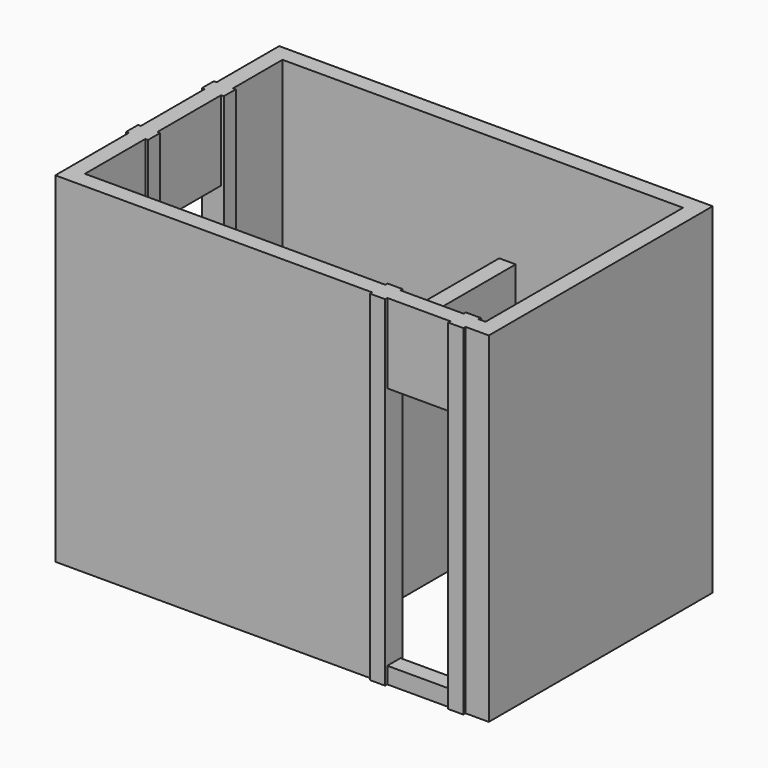
from build123d import *

# Parameters (mm, degrees)
F0_W     = 152.4
F0_H     = 139.7
F0_W_2   = 25.4
F0_W_3   = 139.7
F0_H_2   = 152.4
F0_H_3   = 25.4
F1_DEPTH = 2997.2
F2_START = 2260.6
F0_H_4   = 736.6
F0_W_4   = 584.2
F2_DEPTH = 736.6
F0_H_5   = 2286
F3_DEPTH = 152.4
F4_DEPTH = 2032


with BuildPart() as f1:
    # F0 (on Top) → F1 (new body)
    with BuildSketch(Plane.XY):
        Polygon((2006.6, 0), (0, 0), (0, 698.5), (-152.4, 698.5), (-152.4, -152.4), (2781.3, -152.4), (2781.3, 0), (2159, 0), align=None)
        with Locations((-76.2, 768.35)):
            Rectangle(F0_W, F0_H)
        with Locations((12.7, 768.35)):
            Rectangle(F0_W_2, F0_H)
        with Locations((-165.1, 768.35)):
            Rectangle(F0_W_2, F0_H)
        Polygon((2781.3, 25.4), (2781.3, 0), (2921, 0), (2921, 25.4), (2844.8, 25.4), align=None)
        with Locations((2851.15, -76.2)):
            Rectangle(F0_W_3, F0_H_2)
        with Locations((2851.15, -165.1)):
            Rectangle(F0_W_3, F0_H_3)
    extrude(amount=F1_DEPTH)



with BuildPart() as f1b:
    # F0 (on Top) → F1, piece 2 (new body)
    with BuildSketch(Plane.XY):
        Polygon((0, 2286), (2006.6, 2286), (2159, 2286), (3708.4, 2286), (3708.4, 0), (3644.9, 0), (3644.9, -152.4), (3860.8, -152.4), (3860.8, 2438.4), (-152.4, 2438.4), (-152.4, 1714.5), (0, 1714.5), align=None)
        with Locations((-76.2, 1644.65)):
            Rectangle(F0_W, F0_H)
        with Locations((12.7, 1644.65)):
            Rectangle(F0_W_2, F0_H)
        with Locations((-165.1, 1644.65)):
            Rectangle(F0_W_2, F0_H)
        with Locations((3575.05, 12.7)):
            Rectangle(F0_W_3, F0_H_3)
        with Locations((3575.05, -76.2)):
            Rectangle(F0_W_3, F0_H_2)
        with Locations((3575.05, -165.1)):
            Rectangle(F0_W_3, F0_H_3)
    extrude(amount=F1_DEPTH)


with BuildPart() as f1_1:
    add(f1.part)

    add(f1b.part)  # F2 merges F1b
    # F0 (on Top) → F2 (join)
    with BuildSketch(Plane.XY.offset(F2_START)):
        with Locations((-76.2, 1206.5)):
            Rectangle(F0_W, F0_H_4)
        with Locations((3213.1, -76.2)):
            Rectangle(F0_W_4, F0_H_2)
    extrude(amount=F2_DEPTH)

    # F0 (on Top) → F3 (join)
    with BuildSketch(Plane.XY):
        Polygon((2006.6, 0), (0, 0), (0, 698.5), (-152.4, 698.5), (-152.4, -152.4), (2781.3, -152.4), (2781.3, 0), (2159, 0), align=None)
        with Locations((2082.8, 1143)):
            Rectangle(F0_W, F0_H_5)
        with Locations((-76.2, 768.35)):
            Rectangle(F0_W, F0_H)
        with Locations((12.7, 768.35)):
            Rectangle(F0_W_2, F0_H)
        Polygon((0, 2286), (2006.6, 2286), (2159, 2286), (3708.4, 2286), (3708.4, 0), (3644.9, 0), (3644.9, -152.4), (3860.8, -152.4), (3860.8, 2438.4), (-152.4, 2438.4), (-152.4, 1714.5), (0, 1714.5), align=None)
        with Locations((-76.2, 1206.5)):
            Rectangle(F0_W, F0_H_4)
        with Locations((-165.1, 768.35)):
            Rectangle(F0_W_2, F0_H)
        Polygon((2781.3, 25.4), (2781.3, 0), (2921, 0), (2921, 25.4), (2844.8, 25.4), align=None)
        with Locations((2851.15, -76.2)):
            Rectangle(F0_W_3, F0_H_2)
        with Locations((-76.2, 1644.65)):
            Rectangle(F0_W, F0_H)
        with Locations((12.7, 1644.65)):
            Rectangle(F0_W_2, F0_H)
        with Locations((3213.1, -76.2)):
            Rectangle(F0_W_4, F0_H_2)
        with Locations((2851.15, -165.1)):
            Rectangle(F0_W_3, F0_H_3)
        with Locations((-165.1, 1644.65)):
            Rectangle(F0_W_2, F0_H)
        with Locations((3575.05, 12.7)):
            Rectangle(F0_W_3, F0_H_3)
        with Locations((3575.05, -76.2)):
            Rectangle(F0_W_3, F0_H_2)
        with Locations((3575.05, -165.1)):
            Rectangle(F0_W_3, F0_H_3)
    extrude(amount=-F3_DEPTH)

    # F0 (on Top) → F4 (join)
    with BuildSketch(Plane.XY):
        with Locations((2082.8, 1143)):
            Rectangle(F0_W, F0_H_5)
    extrude(amount=F4_DEPTH)


solid = f1_1.part
